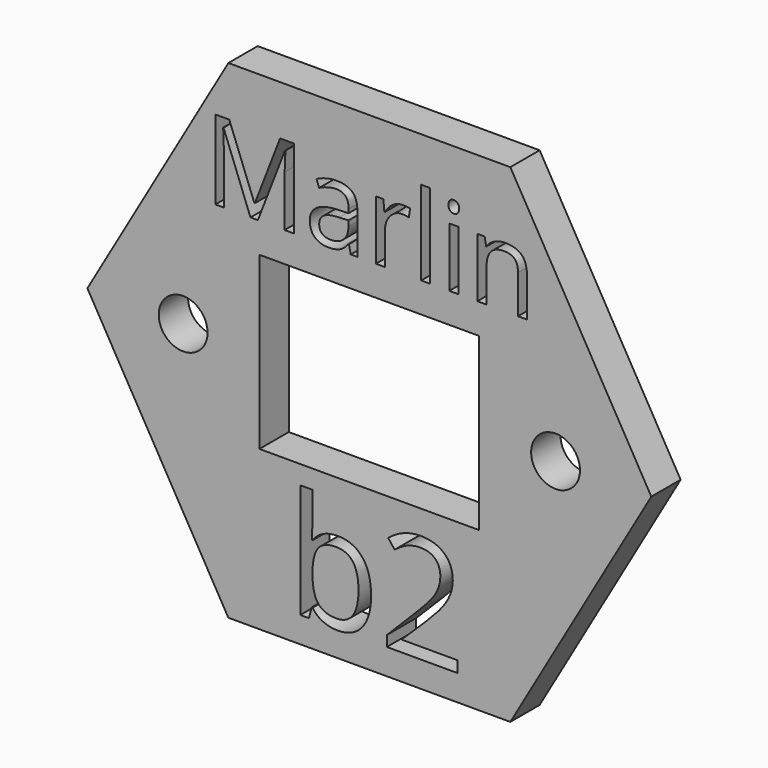
from build123d import *

# Parameters (mm, degrees)
F0_R         = 2
F0_W         = 18
F0_H         = 14
F1_DEPTH     = 3
F2_TEXT_SIZE = 9.0870845604
F3_DEPTH     = 25
F4_TEXT_SIZE = 12.3081677076
F5_DEPTH     = 25


# Not quite as in the source:
# - Text() gives the source's letters only with a copy of the font that has no kerning and outlines rounded to 1/6400 em; it was checked with that copy


with BuildPart() as f1:
    # F0 (on Front) → F1 (new body)
    with BuildSketch(Plane.XZ):
        Polygon((-11.5470053838, -20), (11.5470053838, -20), (23.0940107676, 0), (11.5470053838, 20), (-11.5470053838, 20), (-23.0940107676, 0), align=None)
        with Locations((-15.25, 0)):
            Circle(F0_R, mode=Mode.SUBTRACT)
        Rectangle(F0_W, F0_H, mode=Mode.SUBTRACT)
        with Locations((15.25, 0)):
            Circle(F0_R, mode=Mode.SUBTRACT)
    extrude(amount=F1_DEPTH)

    # F2 (on face) → F3 (cut)
    with BuildSketch(Plane.XZ.offset(3)):
        with Locations((-13.5, 9.4553306832)):
            Text('Marlin', F2_TEXT_SIZE, font='Open Sans', text_align=(TextAlign.LEFT, TextAlign.BOTTOM))
    extrude(amount=-F3_DEPTH, mode=Mode.SUBTRACT)

    # F4 (on face) → F5 (cut)
    with BuildSketch(Plane.XZ.offset(3)):
        with Locations((-6.7138727754, -17.8846810013)):
            Text('b2', F4_TEXT_SIZE, font='Open Sans', text_align=(TextAlign.LEFT, TextAlign.BOTTOM))
    extrude(amount=-F5_DEPTH, mode=Mode.SUBTRACT)


solid = f1.part
